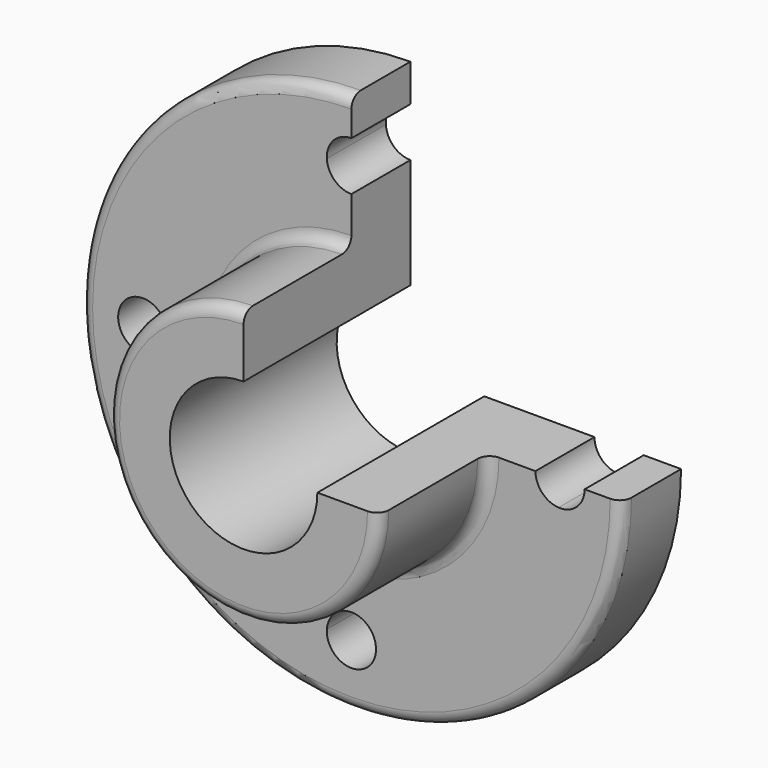
from build123d import *

# Parameters (mm, degrees)
F0_R     = 35.052
F0_R_2   = 19.05
F1_DEPTH = 53.848
F0_R_3   = 69.85
F2_DEPTH = 19.05
F3_W     = 73.3096525073
F3_H     = 72.7184489369
F4_DEPTH = 222
F5_W     = 74.8862102628
F5_H     = 75.4774138331
F6_DEPTH = 53.849
F7_R     = 3.048


# Not quite as in the source:
# - an extrude ends at something that could not be found from the text; its depth is read off the source's solid


with BuildPart() as f1:
    # F0 (on Front) → F1 (new body)
    with BuildSketch(Plane.XZ):
        Circle(F0_R)
        Circle(F0_R_2, mode=Mode.SUBTRACT)
    extrude(amount=F1_DEPTH)

    # F0 (on Front) → F2 (join)
    with BuildSketch(Plane.XZ):
        Circle(F0_R_3)
        with BuildLine():
            ThreePointArc((6.3389523479, 53.4735896226), (38.0762859533, 38.0762859533), (53.4735896226, 6.3389523479))
            ThreePointArc((53.4735896226, 6.3389523479), (58.2037429965, 4.6206063399), (60.198, 0))
            ThreePointArc((60.198, 0), (58.2037429965, -4.6206063399), (53.4735896226, -6.3389523479))
            ThreePointArc((53.4735896226, -6.3389523479), (38.0762859533, -38.0762859533), (6.3389523479, -53.4735896226))
            ThreePointArc((6.3389523479, -53.4735896226), (6.3472374861, -53.6607133338), (6.35, -53.848))
            ThreePointArc((6.35, -53.848), (-0.1872866662, -60.1952374861), (-6.3389523479, -53.4735896226))
            ThreePointArc((-6.3389523479, -53.4735896226), (-38.0762859533, -38.0762859533), (-53.4735896226, -6.3389523479))
            ThreePointArc((-53.4735896226, -6.3389523479), (-60.198, 0), (-53.4735896226, 6.3389523479))
            ThreePointArc((-53.4735896226, 6.3389523479), (-38.0762859533, 38.0762859533), (-6.3389523479, 53.4735896226))
            ThreePointArc((-6.3389523479, 53.4735896226), (-0.1872866662, 60.1952374861), (6.35, 53.848))
            ThreePointArc((6.35, 53.848), (6.3472374861, 53.6607133338), (6.3389523479, 53.4735896226))
        make_face(mode=Mode.SUBTRACT)
        with BuildLine():
            ThreePointArc((53.4735896226, -6.3389523479), (47.498, 0), (53.4735896226, 6.3389523479))
            ThreePointArc((53.4735896226, 6.3389523479), (38.0762859533, 38.0762859533), (6.3389523479, 53.4735896226))
            ThreePointArc((6.3389523479, 53.4735896226), (0, 47.498), (-6.3389523479, 53.4735896226))
            ThreePointArc((-6.3389523479, 53.4735896226), (-38.0762859533, 38.0762859533), (-53.4735896226, 6.3389523479))
            ThreePointArc((-53.4735896226, 6.3389523479), (-49.2273936601, 4.3557429965), (-47.498, 0))
            ThreePointArc((-47.498, 0), (-49.2273936601, -4.3557429965), (-53.4735896226, -6.3389523479))
            ThreePointArc((-53.4735896226, -6.3389523479), (-38.0762859533, -38.0762859533), (-6.3389523479, -53.4735896226))
            ThreePointArc((-6.3389523479, -53.4735896226), (0, -47.498), (6.3389523479, -53.4735896226))
            ThreePointArc((6.3389523479, -53.4735896226), (38.0762859533, -38.0762859533), (53.4735896226, -6.3389523479))
        make_face()
        Circle(F0_R, mode=Mode.SUBTRACT)
    extrude(amount=F2_DEPTH)

    # F3 (on Front) → F4 (cut, through all)
    with BuildSketch(Plane.XZ):
        with Locations((36.6548262537, 36.3592244685)):
            Rectangle(F3_W, F3_H)
    extrude(amount=-F4_DEPTH, mode=Mode.SUBTRACT)

    # F5 (on Front) → F6 (cut, through all)
    with BuildSketch(Plane.XZ):
        with Locations((37.4431051314, 37.7387069166)):
            Rectangle(F5_W, F5_H)
    extrude(amount=F6_DEPTH, mode=Mode.SUBTRACT)

    # F7
    f7_edges = [f1.edges().sort_by_distance(p)[0] for p in [
        (-24.785507, -53.848, -24.785507),
        (-24.785507, -19.05, -24.785507),
        (-49.391409, -19.05, -49.391409),
    ]]
    fillet(f7_edges, radius=F7_R)


solid = f1.part
